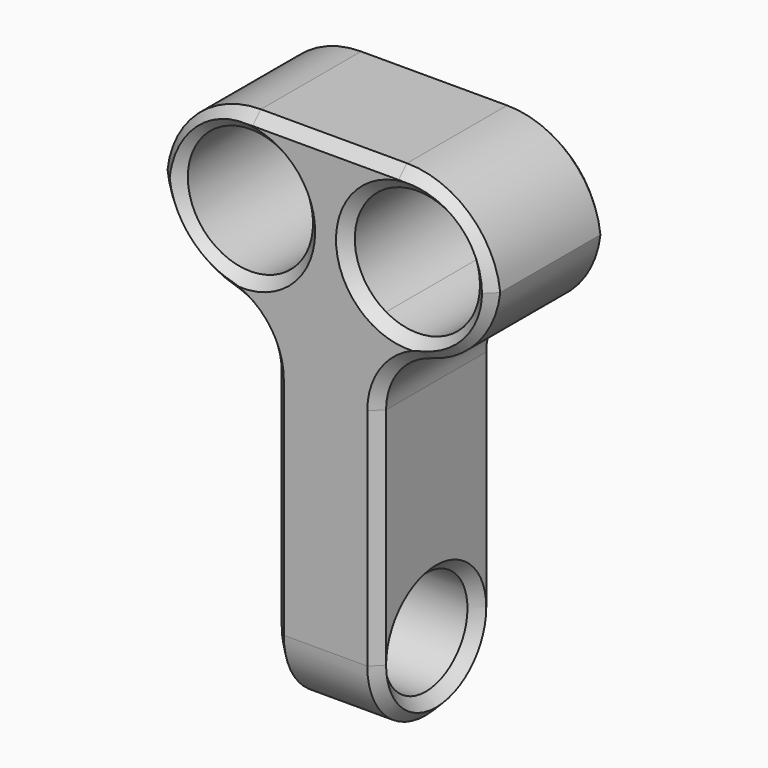
from build123d import *

# Parameters (mm, degrees)
F0_W         = 5
F0_H         = 17
F1_DEPTH     = 7
F3_D         = 5
F4_T1_DEPTH  = 29.5
F5_R         = 3.49999
F6_R         = 3
F7_T1_DEPTH  = 10.7715938526
F7_T3_DEPTH  = 7
F7_T5_DEPTH  = 2e-05
F7_T16_ANGLE = 74.5339900582
F7_T18_ANGLE = 117.281460121
F7_T20_ANGLE = 132.7531885059
F7_T22_ANGLE = 74.5339900582
F7_T24_ANGLE = 117.281460121
F7_T26_ANGLE = 132.7531885059
F7_T28_ANGLE = 90
F7_T30_ANGLE = 90
F7_T34_ANGLE = 74.5339900582
F7_T36_ANGLE = 90
F7_T38_ANGLE = 117.281460121
F7_T40_ANGLE = 90
F7_T44_ANGLE = 132.7531885059
F7_T46_ANGLE = 74.5339900582
F7_T48_ANGLE = 117.281460121
F7_T50_ANGLE = 132.7531885059


# Not quite as in the source:
# - a fillet or chamfer that OpenCascade refuses, or shapes differently, is made with other operations: its cross-section is extruded or revolved along the edge and cut away or added
# - two fillets or chamfers of one size are made in one step
# - a fillet or chamfer is up to 0.001 mm smaller than in the source, because OpenCascade refuses the exact size


with BuildPart() as f1:
    # F0 (on Front) → F1 (new body)
    with BuildSketch(Plane.XZ):
        with BuildLine():
            Line((8, 12.5), (2.5, 12.5))
            Line((2.5, 12.5), (2.5, 11.0980762114))
            ThreePointArc((2.5, 11.0980762114), (5.5, 11.0980762114), (7, 8.5))
            ThreePointArc((7, 8.5), (5.5, 5.9019237886), (2.5, 5.9019237886))
            Line((2.5, 5.9019237886), (2.5, 4.5))
            Line((2.5, 4.5), (8, 4.5))
            Line((8, 4.5), (8, 12.5))
        make_face()
        with BuildLine():
            Line((-2.5, 11.0980762114), (-2.5, 12.5))
            Line((-2.5, 12.5), (-8, 12.5))
            Line((-8, 12.5), (-8, 4.5))
            Line((-8, 4.5), (-2.5, 4.5))
            Line((-2.5, 4.5), (-2.5, 5.9019237886))
            ThreePointArc((-2.5, 5.9019237886), (-7, 8.5), (-2.5, 11.0980762114))
        make_face()
        with BuildLine():
            Line((2.5, 11.0980762114), (2.5, 12.5))
            Line((2.5, 12.5), (-2.5, 12.5))
            Line((-2.5, 12.5), (-2.5, 11.0980762114))
            ThreePointArc((-2.5, 11.0980762114), (-1.4019237886, 10), (-1, 8.5))
            ThreePointArc((-1, 8.5), (-1.4019237886, 7), (-2.5, 5.9019237886))
            Line((-2.5, 5.9019237886), (-2.5, 4.5))
            Line((-2.5, 4.5), (2.5, 4.5))
            Line((2.5, 4.5), (2.5, 5.9019237886))
            ThreePointArc((2.5, 5.9019237886), (1, 8.5), (2.5, 11.0980762114))
        make_face()
        with Locations((0, -4)):
            Rectangle(F0_W, F0_H)
    extrude(amount=F1_DEPTH)

    # F3 (through all)
    with Locations(Plane.YZ.offset(2.5)):
        with Locations((-3.5, -9)):
            Hole(F3_D / 2)

    # F4: fillet of radius 4.5 on 4 edges, made by hand

    # F4_s2 → F4_t1 (cut)
    with BuildSketch(Plane.XZ.offset(-11.25)):
        with BuildLine():
            ThreePointArc((3.5, 12.5), (6.6819805153, 11.1819805153), (8, 8))
            Line((8, 8), (8, 12.5))
            Line((8, 12.5), (3.5, 12.5))
        make_face()
        with BuildLine():
            ThreePointArc((-3.5, 12.5), (-6.6819805153, 11.1819805153), (-8, 8))
            Line((-8, 8), (-8, 12.5))
            Line((-8, 12.5), (-3.5, 12.5))
        make_face()
        with BuildLine():
            ThreePointArc((8, 9), (6.6819805153, 5.8180194847), (3.5, 4.5))
            Line((3.5, 4.5), (8, 4.5))
            Line((8, 4.5), (8, 9))
        make_face()
        with BuildLine():
            ThreePointArc((-8, 9), (-6.6819805153, 5.8180194847), (-3.5, 4.5))
            Line((-3.5, 4.5), (-8, 4.5))
            Line((-8, 4.5), (-8, 9))
        make_face()
    extrude(amount=F4_T1_DEPTH, mode=Mode.SUBTRACT)

    # F5 (radius 3.5 in the source; OpenCascade refuses exactly that, so slightly less here)
    f5_edges = [f1.edges().sort_by_distance(p)[0] for p in [
        (0, 0, -12.5),
        (0, -7, -12.5),
    ]]
    fillet(f5_edges, radius=F5_R)

    # F6
    f6_edges = [f1.edges().sort_by_distance(p)[0] for p in [
        (2.5, -3.5, 4.5),
        (-2.5, -3.5, 4.5),
    ]]
    fillet(f6_edges, radius=F6_R)

    # F7: chamfer of 0.5 on 30 edges, made by hand

    # F7_s2 → F7_t1 (cut)
    with BuildSketch(Plane.XY.offset(-9.00001)):
        Polygon((2, 0), (2.5, -0.5), (2.5, 0), align=None)
        Polygon((-2, 0), (-2.5, -0.5), (-2.5, 0), align=None)
        Polygon((2.5, -6.5), (2, -7), (2.5, -7), align=None)
        Polygon((-2.5, -6.5), (-2, -7), (-2.5, -7), align=None)
    extrude(amount=F7_T1_DEPTH, mode=Mode.SUBTRACT)

    # F7_s4 → F7_t3 (cut)
    with BuildSketch(Plane.YZ.offset(-3.5)):
        Polygon((0, 12), (-0.5, 12.5), (0, 12.5), align=None)
        Polygon((-6.5, 12.5), (-7, 12), (-7, 12.5), align=None)
    extrude(amount=F7_T3_DEPTH, mode=Mode.SUBTRACT)

    # F7_s6 → F7_t5 (cut)
    with BuildSketch(Plane.XZ.offset(3.49999)):
        Polygon((2.5, -12), (2, -12.5), (2.5, -12.5), align=None)
        Polygon((-2.5, -12), (-2, -12.5), (-2.5, -12.5), align=None)
    extrude(amount=F7_T5_DEPTH, mode=Mode.SUBTRACT)

    # F7_s7 → F7_t8 (revolve, cut)
    with BuildSketch(Plane.XY.offset(8.5)):
        Polygon((-1, -6.5), (-0.5, -7), (-1, -7), align=None)
    revolve(axis=Axis((-4, -7, 8.5), (0, 1, 0)), mode=Mode.SUBTRACT)

    # F7_s9 → F7_t10 (revolve, cut)
    with BuildSketch(Plane(origin=(-0.6806079661, 0, 0.3929491924), x_dir=(0, 1, 0), z_dir=(0.8660254038, 0, -0.5))):
        Polygon((-6.5, 6.3612159322), (-7, 5.8612159322), (-7, 6.3612159322), align=None)
    revolve(axis=Axis((4, -7, 8.5), (0, 1, 0)), mode=Mode.SUBTRACT)

    # F7_s11 → F7_t12 (revolve, cut)
    with BuildSketch(Plane.XY.offset(8.5)):
        Polygon((-0.5, 0), (-1, -0.5), (-1, 0), align=None)
    revolve(axis=Axis((-4, 0, 8.5), (0, 1, 0)), mode=Mode.SUBTRACT)

    # F7_s13 → F7_t14 (revolve, cut)
    with BuildSketch(Plane(origin=(-0.6806079661, 0, 0.3929491924), x_dir=(0, 1, 0), z_dir=(0.8660254038, 0, -0.5))):
        Polygon((0, 5.8612159322), (-0.5, 6.3612159322), (0, 6.3612159322), align=None)
    revolve(axis=Axis((4, 0, 8.5), (0, 1, 0)), mode=Mode.SUBTRACT)

    # F7_s15 → F7_t16 (revolve, cut)
    with BuildSketch(Plane.XY.offset(1.771583853)):
        Polygon((2, 0), (2.5000000001, -0.5), (2.5, 0), align=None)
    revolve(axis=Axis((5.4999999996, 0, 1.771583853), (0, 1, 0)), revolution_arc=F7_T16_ANGLE, mode=Mode.SUBTRACT)

    # F7_s17 → F7_t18 (revolve, cut)
    with BuildSketch(Plane(origin=(-2.8735542897, 0, 3.1088689023), x_dir=(0, 1, 0), z_dir=(-0.6787683205, 0, 0.7343524815))):
        Polygon((0, -12.6791485698), (-0.5, -13.1791485698), (0, -13.1791485698), align=None)
    revolve(axis=Axis((3.4999999999, 0, 9.0000000001), (0, 1, 0)), revolution_arc=F7_T18_ANGLE, mode=Mode.SUBTRACT)

    # F7_s19 → F7_t20 (revolve, cut)
    with BuildSketch(Plane.YZ.offset(3.4999999999)):
        Polygon((0, 12), (-0.5, 12.5), (0, 12.5), align=None)
    revolve(axis=Axis((3.4999999999, 0, 7.9999999999), (0, 1, 0)), revolution_arc=F7_T20_ANGLE, mode=Mode.SUBTRACT)

    # F7_s21 → F7_t22 (revolve, cut)
    with BuildSketch(Plane.XY.offset(1.771583853)):
        Polygon((-2, 0), (-2.5000000001, -0.5), (-2.5, 0), align=None)
    revolve(axis=Axis((-5.4999999996, 0, 1.771583853), (0, -1, 0)), revolution_arc=F7_T22_ANGLE, mode=Mode.SUBTRACT)

    # F7_s23 → F7_t24 (revolve, cut)
    with BuildSketch(Plane(origin=(-5.5642042783, 0, 1.5395362318), x_dir=(0, 1, 0), z_dir=(0.9637888196, 0, -0.2666666667))):
        Polygon((0, 3.7407660435), (-0.5, 3.2407660435), (0, 3.2407660435), align=None)
    revolve(axis=Axis((-3.4999999999, 0, 9.0000000001), (0, 1, 0)), revolution_arc=F7_T24_ANGLE, mode=Mode.SUBTRACT)

    # F7_s25 → F7_t26 (revolve, cut)
    with BuildSketch(Plane(origin=(-5.6005949978, 0, 6.0580131587), x_dir=(0, 1, 0), z_dir=(0.6788416095, 0, -0.7342847331))):
        Polygon((0, -1.1392636899), (-0.5, -1.6392636899), (0, -1.6392636899), align=None)
    revolve(axis=Axis((-3.4999999999, 0, 7.9999999999), (0, 1, 0)), revolution_arc=F7_T26_ANGLE, mode=Mode.SUBTRACT)

    # F7_s27 → F7_t28 (revolve, cut)
    with BuildSketch(Plane.XY.offset(-9.00001)):
        Polygon((2.5, -0.5), (2, 0), (2.5, 0), align=None)
    revolve(axis=Axis((2.5, -3.49999, -9.00001), (-1, 0, 0)), revolution_arc=F7_T28_ANGLE, mode=Mode.SUBTRACT)

    # F7_s29 → F7_t30 (revolve, cut)
    with BuildSketch(Plane.XY.offset(-9.00001)):
        Polygon((2.5, -6.5), (2, -7), (2.5, -7), align=None)
    revolve(axis=Axis((2.5, -3.50001, -9.00001), (1, 0, 0)), revolution_arc=F7_T30_ANGLE, mode=Mode.SUBTRACT)

    # F7_s31 → F7_t32 (revolve, cut)
    with BuildSketch(Plane.XY.offset(-9)):
        Polygon((2.5, -0.5), (2, -1), (2.5, -1), align=None)
    revolve(axis=Axis((2.5, -3.5, -9), (1, 0, 0)), mode=Mode.SUBTRACT)

    # F7_s33 → F7_t34 (revolve, cut)
    with BuildSketch(Plane.XY.offset(1.771583853)):
        Polygon((2.5000000001, -6.5), (2, -7), (2.5, -7), align=None)
    revolve(axis=Axis((5.4999999996, -7, 1.771583853), (0, 1, 0)), revolution_arc=F7_T34_ANGLE, mode=Mode.SUBTRACT)

    # F7_s35 → F7_t36 (revolve, cut)
    with BuildSketch(Plane.XY.offset(-9.00001)):
        Polygon((-2, 0), (-2.5, -0.5), (-2.5, 0), align=None)
    revolve(axis=Axis((-2.5, -3.49999, -9.00001), (-1, 0, 0)), revolution_arc=F7_T36_ANGLE, mode=Mode.SUBTRACT)

    # F7_s37 → F7_t38 (revolve, cut)
    with BuildSketch(Plane(origin=(-2.8735542897, 0, 3.1088689023), x_dir=(0, 1, 0), z_dir=(-0.6787683205, 0, 0.7343524815))):
        Polygon((-6.5, -13.1791485698), (-7, -12.6791485698), (-7, -13.1791485698), align=None)
    revolve(axis=Axis((3.4999999999, -7, 9.0000000001), (0, 1, 0)), revolution_arc=F7_T38_ANGLE, mode=Mode.SUBTRACT)

    # F7_s39 → F7_t40 (revolve, cut)
    with BuildSketch(Plane.XY.offset(-9.00001)):
        Polygon((-2.5, -6.5), (-2, -7), (-2.5, -7), align=None)
    revolve(axis=Axis((-2.5, -3.50001, -9.00001), (1, 0, 0)), revolution_arc=F7_T40_ANGLE, mode=Mode.SUBTRACT)

    # F7_s41 → F7_t42 (revolve, cut)
    with BuildSketch(Plane.XY.offset(-9)):
        Polygon((-2.5, -0.5), (-2, -1), (-2.5, -1), align=None)
    revolve(axis=Axis((-2.5, -3.5, -9), (1, 0, 0)), mode=Mode.SUBTRACT)

    # F7_s43 → F7_t44 (revolve, cut)
    with BuildSketch(Plane.YZ.offset(3.4999999999)):
        Polygon((-6.5, 12.5), (-7, 12), (-7, 12.5), align=None)
    revolve(axis=Axis((3.4999999999, -7, 7.9999999999), (0, 1, 0)), revolution_arc=F7_T44_ANGLE, mode=Mode.SUBTRACT)

    # F7_s45 → F7_t46 (revolve, cut)
    with BuildSketch(Plane.XY.offset(1.771583853)):
        Polygon((-2.5000000001, -6.5), (-2, -7), (-2.5, -7), align=None)
    revolve(axis=Axis((-5.4999999996, -7, 1.771583853), (0, -1, 0)), revolution_arc=F7_T46_ANGLE, mode=Mode.SUBTRACT)

    # F7_s47 → F7_t48 (revolve, cut)
    with BuildSketch(Plane(origin=(-5.5642042783, 0, 1.5395362318), x_dir=(0, 1, 0), z_dir=(0.9637888196, 0, -0.2666666667))):
        Polygon((-6.5, 3.2407660435), (-7, 3.7407660435), (-7, 3.2407660435), align=None)
    revolve(axis=Axis((-3.4999999999, -7, 9.0000000001), (0, 1, 0)), revolution_arc=F7_T48_ANGLE, mode=Mode.SUBTRACT)

    # F7_s49 → F7_t50 (revolve, cut)
    with BuildSketch(Plane(origin=(-5.6005949978, 0, 6.0580131587), x_dir=(0, 1, 0), z_dir=(0.6788416095, 0, -0.7342847331))):
        Polygon((-6.5, -1.6392636899), (-7, -1.1392636899), (-7, -1.6392636899), align=None)
    revolve(axis=Axis((-3.4999999999, -7, 7.9999999999), (0, 1, 0)), revolution_arc=F7_T50_ANGLE, mode=Mode.SUBTRACT)


solid = f1.part
